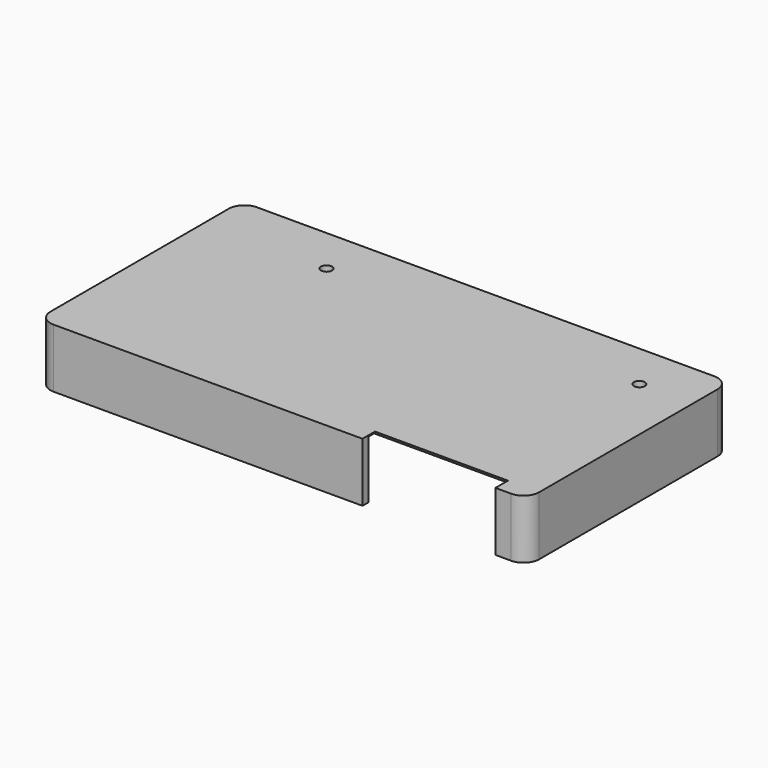
from build123d import *

# Parameters (mm, degrees)
F0_W         = 158.75
F0_H         = 82.55
F1_DEPTH     = 19.177
F2_T         = -2.54
F3_R         = 5.08
F5_D         = 3.556
F6_W         = 43.18
F6_H         = 19.177
F7_DEPTH     = 5.08
F8_T1_DEPTH  = 43.18
F8_T3_DEPTH  = 2.54
F8_T9_DEPTH  = 13.5385226281
F8_T13_DEPTH = 54.1785226281
F8_T20_DEPTH = 13.5385226281
F8_T24_DEPTH = 54.1785226281


# Not quite as in the source:
# - a fillet or chamfer that OpenCascade refuses, or shapes differently, is made with other operations: its cross-section is extruded or revolved along the edge and cut away or added


with BuildPart() as f1:
    # F0 (on Top) → F1 (new body)
    with BuildSketch(Plane.XY):
        with Locations((147.5038135648, 4.0233785152)):
            Rectangle(F0_W, F0_H)
    extrude(amount=F1_DEPTH)

    # F2
    f2_openings = [f1.faces().sort_by_distance(p)[0] for p in [
        (147.503814, 4.023379, 0),
    ]]
    offset(amount=F2_T, openings=f2_openings)

    # F3
    f3_edges = [f1.edges().sort_by_distance(p)[0] for p in [
        (226.878814, -37.251621, 9.5885),
        (226.878814, 45.298379, 9.5885),
        (68.128814, 45.298379, 9.5885),
        (68.128814, -37.251621, 9.5885),
    ]]
    fillet(f3_edges, radius=F3_R)

    # F5 (through all)
    with Locations(Plane.XY.offset(19.177)):
        with Locations((108.0068135648, 30.0583785152), (209.6068135648, 30.0583785152)):
            Hole(F5_D / 2)

    # F6 (on face) → F7 (cut)
    with BuildSketch(Plane.XZ.offset(37.2516214848)):
        with Locations((195.1288135648, 9.5885)):
            Rectangle(F6_W, F6_H)
    extrude(amount=-F7_DEPTH, mode=Mode.SUBTRACT)

    # F8: fillet of radius 5.08 on 3 edges, made by hand

    # F8_s2 → F8_t1 (cut)
    with BuildSketch(Plane.YZ.offset(173.5388135648)):
        with BuildLine():
            ThreePointArc((-32.1716214848, 19.177), (-30.3122124335, 17.3175909488), (-27.7722124335, 16.637))
            Line((-27.7722124335, 16.637), (-27.7722124335, 16.5354))
            Line((-27.7722124335, 16.5354), (-32.1716214848, 16.5354))
            Line((-32.1716214848, 16.5354), (-32.2732214848, 16.637))
            ThreePointArc((-32.2732214848, 16.637), (-32.2732214848, 17.907), (-32.2596096658, 19.1262))
            Line((-32.2596096658, 19.1262), (-32.1716214848, 19.177))
        make_face()
    extrude(amount=F8_T1_DEPTH, mode=Mode.SUBTRACT)

    # F8_s4 → F8_t3 (cut)
    with BuildSketch(Plane.XZ.offset(32.1716214848)):
        with BuildLine():
            ThreePointArc((173.5388135648, 19.177), (171.6794045136, 17.3175909488), (169.1394045136, 16.637))
            Line((169.1394045136, 16.637), (169.1394045136, 16.5354))
            Line((169.1394045136, 16.5354), (173.5388135648, 16.5354))
            Line((173.5388135648, 16.5354), (173.6404135648, 16.637))
            ThreePointArc((173.6404135648, 16.637), (173.6404135648, 17.907), (173.6268017458, 19.1262))
            Line((173.6268017458, 19.1262), (173.5388135648, 19.177))
        make_face()
        with BuildLine():
            ThreePointArc((216.7188135648, 19.177), (218.578222616, 17.3175909488), (221.118222616, 16.637))
            Line((221.118222616, 16.637), (221.118222616, 16.5354))
            Line((221.118222616, 16.5354), (216.7188135648, 16.5354))
            Line((216.7188135648, 16.5354), (216.6172135648, 16.637))
            ThreePointArc((216.6172135648, 16.637), (216.6172135648, 17.907), (216.6308253838, 19.1262))
            Line((216.6308253838, 19.1262), (216.7188135648, 19.177))
        make_face()
    extrude(amount=F8_T3_DEPTH, mode=Mode.SUBTRACT)


with BuildPart() as f8_tool7:
    # F8_s8 → F8_t9 (new body)
    with BuildSketch(Plane.XZ.offset(21.1730988567)):
        with BuildLine():
            ThreePointArc((173.5388135648, 19.177), (171.6794045136, 17.3175909488), (169.1394045136, 16.637))
            Line((169.1394045136, 16.637), (169.1394045136, 16.5354))
            Line((169.1394045136, 16.5354), (173.5388135648, 16.5354))
            Line((173.5388135648, 16.5354), (173.6404135648, 16.637))
            ThreePointArc((173.6404135648, 16.637), (173.6404135648, 17.907), (173.6268017458, 19.1262))
            Line((173.6268017458, 19.1262), (173.5388135648, 19.177))
        make_face()
    extrude(amount=F8_T9_DEPTH)

    split(bisect_by=Plane.XZ.offset(32.1716214848), keep=Keep.BOTTOM)


with BuildPart() as f8_tool11:
    # F8_s12 → F8_t13 (new body)
    with BuildSketch(Plane.YZ.offset(162.5402909367)):
        with BuildLine():
            ThreePointArc((-32.1716214848, 19.177), (-30.3122124335, 17.3175909488), (-27.7722124335, 16.637))
            Line((-27.7722124335, 16.637), (-27.7722124335, 16.5354))
            Line((-27.7722124335, 16.5354), (-32.1716214848, 16.5354))
            Line((-32.1716214848, 16.5354), (-32.2732214848, 16.637))
            ThreePointArc((-32.2732214848, 16.637), (-32.2732214848, 17.907), (-32.2596096658, 19.1262))
            Line((-32.2596096658, 19.1262), (-32.1716214848, 19.177))
        make_face()
    extrude(amount=F8_T13_DEPTH)

    split(bisect_by=Plane.YZ.offset(173.5388135648), keep=Keep.BOTTOM)


with BuildPart() as f8_tool7_1:
    add(f8_tool7.part)

    # F8_t15: intersect F8_tool11
    add(f8_tool11.part, mode=Mode.INTERSECT)


with BuildPart() as f1_1:
    add(f1.part)

    # F8_t5: cut F8_tool7
    add(f8_tool7_1.part, mode=Mode.SUBTRACT)


with BuildPart() as f8_tool18:
    # F8_s19 → F8_t20 (new body)
    with BuildSketch(Plane.XZ.offset(34.7116214848)):
        with BuildLine():
            ThreePointArc((216.7188135648, 19.177), (218.578222616, 17.3175909488), (221.118222616, 16.637))
            Line((221.118222616, 16.637), (221.118222616, 16.5354))
            Line((221.118222616, 16.5354), (216.7188135648, 16.5354))
            Line((216.7188135648, 16.5354), (216.6172135648, 16.637))
            ThreePointArc((216.6172135648, 16.637), (216.6172135648, 17.907), (216.6308253838, 19.1262))
            Line((216.6308253838, 19.1262), (216.7188135648, 19.177))
        make_face()
    extrude(amount=-F8_T20_DEPTH)

    split(bisect_by=Plane.XZ.offset(32.1716214848), keep=Keep.BOTTOM)


with BuildPart() as f8_tool22:
    # F8_s23 → F8_t24 (new body)
    with BuildSketch(Plane.YZ.offset(173.5388135648)):
        with BuildLine():
            ThreePointArc((-32.1716214848, 19.177), (-30.3122124335, 17.3175909488), (-27.7722124335, 16.637))
            Line((-27.7722124335, 16.637), (-27.7722124335, 16.5354))
            Line((-27.7722124335, 16.5354), (-32.1716214848, 16.5354))
            Line((-32.1716214848, 16.5354), (-32.2732214848, 16.637))
            ThreePointArc((-32.2732214848, 16.637), (-32.2732214848, 17.907), (-32.2596096658, 19.1262))
            Line((-32.2596096658, 19.1262), (-32.1716214848, 19.177))
        make_face()
    extrude(amount=F8_T24_DEPTH)

    split(bisect_by=Plane.YZ.offset(216.7188135648), keep=Keep.TOP)


with BuildPart() as f8_tool18_1:
    add(f8_tool18.part)

    # F8_t26: intersect F8_tool22
    add(f8_tool22.part, mode=Mode.INTERSECT)


with BuildPart() as f1_2:
    add(f1_1.part)

    # F8_t16: cut F8_tool18
    add(f8_tool18_1.part, mode=Mode.SUBTRACT)


solid = f1_2.part
